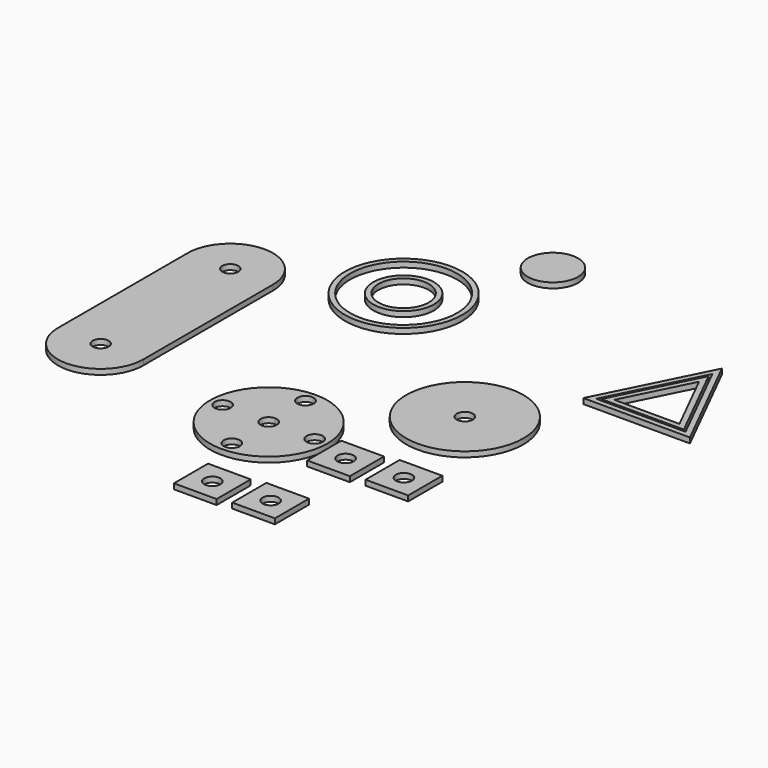
from build123d import *

# Parameters (mm, degrees)
F1_R      = 34.925
F1_R_2    = 4.826
F2_DEPTH  = 3.175
F3_R      = 34.925
F4_DEPTH  = 3.175
F5_R      = 4.826
F6_DEPTH  = 25.4
F7_W      = 25.4
F7_H      = 25.4
F7_R      = 4.826
F8_DEPTH  = 3.175
F0_R      = 18.034
F0_R_2    = 14.986
F9_DEPTH  = 3.175
F0_R_3    = 34.9504
F0_R_4    = 31.877
F10_R     = 4.7625
F11_DEPTH = 3.175
F12_DEPTH = 3.175
F13_DEPTH = 3.175


# Not quite as in the source:
# - a feature names something its author has since deleted; it is built from what else it names


with BuildPart() as f2:
    # F1 (on Top) → F2 (new body)
    with BuildSketch(Plane.XY):
        with Locations((-41.45681113, -107.801027596)):
            Circle(F1_R)
        with Locations((-41.45681113, -135.201277596)):
            Circle(F1_R_2, mode=Mode.SUBTRACT)
        with Locations((-68.85706113, -107.801027596)):
            Circle(F1_R_2, mode=Mode.SUBTRACT)
        with BuildLine():
            ThreePointArc((-41.45681113, -102.975027596), (-38.044313804, -104.38853027), (-36.63081113, -107.801027596))
            ThreePointArc((-36.63081113, -107.801027596), (-38.044313804, -111.213524922), (-41.45681113, -112.627027596))
            ThreePointArc((-41.45681113, -112.627027596), (-46.28281113, -107.801027596), (-41.45681113, -102.975027596))
        make_face(mode=Mode.SUBTRACT)
        with Locations((-14.05656113, -107.801027596)):
            Circle(F1_R_2, mode=Mode.SUBTRACT)
        with Locations((-41.45681113, -80.400777596)):
            Circle(F1_R_2, mode=Mode.SUBTRACT)
    extrude(amount=F2_DEPTH)


with BuildPart() as f4:
    # F3 (on Top) → F4 (new body)
    with BuildSketch(Plane.XY):
        with Locations((26.4654487837, -46.6705858707)):
            Circle(F3_R)
    extrude(amount=F4_DEPTH)

    # F5 (on face) → F6 (cut)
    with BuildSketch(Plane.XY.offset(3.175)):
        with Locations((26.4654487837, -46.6705858707)):
            Circle(F5_R)
    extrude(amount=-F6_DEPTH, mode=Mode.SUBTRACT)


with BuildPart() as f8:
    # F7 (on Top) → F8 (new body)
    with BuildSketch(Plane.XY):
        with Locations((9.4302088464, -114.1496481273)):
            Rectangle(F7_W, F7_H)
        with Locations((9.4302088464, -114.1496481273)):
            Circle(F7_R, mode=Mode.SUBTRACT)
    extrude(amount=F8_DEPTH)

    # F7 (on Top) → F12 (join)
    with BuildSketch(Plane.XY):
        with Locations((9.4302088464, -114.1496481273)):
            Rectangle(F7_W, F7_H)
        with Locations((9.4302088464, -114.1496481273)):
            Circle(F7_R, mode=Mode.SUBTRACT)
    extrude(amount=F12_DEPTH)


with BuildPart() as f9:
    # F0 (on Top) → F9 (new body)
    with BuildSketch(Plane.XY):
        with Locations((-73.4194368124, 32.6004140079)):
            Circle(F0_R)
        with Locations((-73.4194368124, 32.6004140079)):
            Circle(F0_R_2, mode=Mode.SUBTRACT)
    extrude(amount=F9_DEPTH)


with BuildPart() as f9b:
    # F0 (on Top) → F9, piece 2 (new body)
    with BuildSketch(Plane.XY):
        with Locations((-73.4194368124, 32.6004140079)):
            Circle(F0_R_3)
        with Locations((-73.4194368124, 32.6004140079)):
            Circle(F0_R_4, mode=Mode.SUBTRACT)
    extrude(amount=F9_DEPTH)


with BuildPart() as f9c:
    # F0 (on Top) → F9, piece 3 (new body)
    with BuildSketch(Plane.XY):
        Polygon((89.5012710243, 65.8874005459), (57.7512710243, 2.3874005459), (89.5012710243, 2.3874005459), (121.2512710243, 2.3874005459), align=None)
        Polygon((116.1140131101, 5.5624005459), (89.5012710243, 5.5624005459), (62.8885289386, 5.5624005459), (89.5012710243, 58.7878847174), align=None, mode=Mode.SUBTRACT)
    extrude(amount=F9_DEPTH)


with BuildPart() as f9d:
    # F0 (on Top) → F9, piece 4 (new body)
    with BuildSketch(Plane.XY):
        Polygon((89.5012710243, 55.948078386), (64.9434321043, 6.8324005459), (89.5012710243, 6.8324005459), (114.0591099444, 6.8324005459), align=None)
        Polygon((108.9218520301, 10.0074005459), (89.5012710243, 10.0074005459), (70.0806900186, 10.0074005459), (89.5012710243, 48.8485625574), align=None, mode=Mode.SUBTRACT)
    extrude(amount=F9_DEPTH)


with BuildPart() as f11:
    # F10 (on Top) → F11 (new body)
    with BuildSketch(Plane.XY):
        with BuildLine():
            Line((-126.3140311956, -95.0520038605), (-126.3140311956, 1.4679961395))
            ThreePointArc((-126.3140311956, 1.4679961395), (-151.7140311956, 26.8679961395), (-177.1140311956, 1.4679961395))
            Line((-177.1140311956, 1.4679961395), (-177.1140311956, -95.0520038605))
            ThreePointArc((-177.1140311956, -95.0520038605), (-151.7140311956, -120.4520038605), (-126.3140311956, -95.0520038605))
        make_face()
        with Locations((-151.7140311956, -95.0520038605)):
            Circle(F10_R, mode=Mode.SUBTRACT)
        with Locations((-151.7140311956, 1.4679961395)):
            Circle(F10_R, mode=Mode.SUBTRACT)
    extrude(amount=F11_DEPTH)


with BuildPart() as f12:
    # F7 (on Top) → F12, piece 2 (new body)
    with BuildSketch(Plane.XY):
        with Locations((42.7242840971, -112.3598849141)):
            Rectangle(F7_W, F7_H)
        with Locations((42.7242840971, -112.3598849141)):
            Circle(F7_R, mode=Mode.SUBTRACT)
    extrude(amount=F12_DEPTH)


with BuildPart() as f12b:
    # F7 (on Top) → F12, piece 3 (new body)
    with BuildSketch(Plane.XY):
        with Locations((-24.5669036167, -170.8565043216)):
            Rectangle(F7_W, F7_H)
        with Locations((-24.5669036167, -170.8565043216)):
            Circle(F7_R, mode=Mode.SUBTRACT)
    extrude(amount=F12_DEPTH)


with BuildPart() as f12c:
    # F7 (on Top) → F12, piece 4 (new body)
    with BuildSketch(Plane.XY):
        with Locations((8.7271716339, -169.0667411084)):
            Rectangle(F7_W, F7_H)
        with Locations((8.7271716339, -169.0667411084)):
            Circle(F7_R, mode=Mode.SUBTRACT)
    extrude(amount=F12_DEPTH)


with BuildPart() as f13:
    # F0 (on Top) → F13 (new body)
    with BuildSketch(Plane.XY):
        Polygon((89.5012710243, 65.8874005459), (57.7512710243, 2.3874005459), (89.5012710243, 2.3874005459), (121.2512710243, 2.3874005459), align=None)
        Polygon((116.1140131101, 5.5624005459), (89.5012710243, 5.5624005459), (62.8885289386, 5.5624005459), (89.5012710243, 58.7878847174), align=None, mode=Mode.SUBTRACT)
    extrude(amount=F13_DEPTH)


with BuildPart() as f13b:
    # F0 (on Top) → F13, piece 2 (new body)
    with BuildSketch(Plane.XY):
        with Locations((-73.4194368124, 32.6004140079)):
            Circle(F0_R_3)
        with Locations((-73.4194368124, 32.6004140079)):
            Circle(F0_R_4, mode=Mode.SUBTRACT)
    extrude(amount=F13_DEPTH)


with BuildPart() as f13c:
    # F0 (on Top) → F13, piece 3 (new body)
    with BuildSketch(Plane.XY):
        with Locations((-35.3792831302, 96.1990430951)):
            Circle(F0_R_2)
    extrude(amount=F13_DEPTH)


solid = Compound([f2.part, f4.part, f8.part, f9.part, f9b.part, f9c.part, f9d.part, f11.part, f12.part, f12b.part, f12c.part, f13.part, f13b.part, f13c.part])
